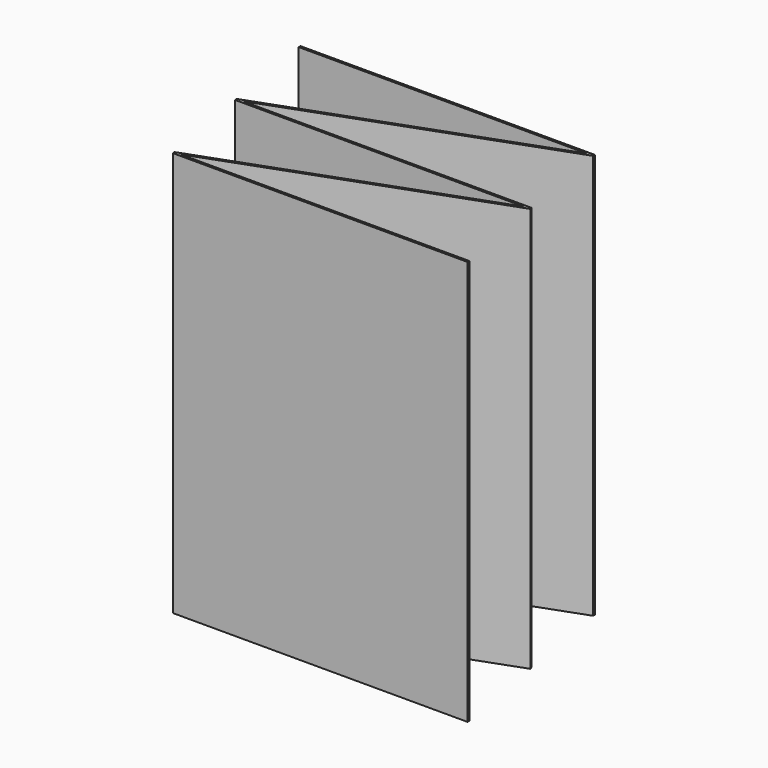
from build123d import *

# Parameters (mm, degrees)
F0_W     = 80
F0_H     = 110
F1_DEPTH = 0.6
F2_COUNT = 2
F2_ANGLE = 20
F3_COUNT = 2
F3_ANGLE = 20
F4_COUNT = 2
F4_ANGLE = 20
F5_COUNT = 2
F5_ANGLE = 20


with BuildPart() as f1:
    # F0 (on Front) → F1 (new body)
    with BuildSketch(Plane.XZ):
        Rectangle(F0_W, F0_H)
    extrude(amount=F1_DEPTH)


with BuildPart() as f2_1:
    # F2: instance of F1
    add(f1.part.rotate(Axis((-40, -0.6, 0), (0, 0, 1)), 1 * F2_ANGLE / (F2_COUNT - 1)))


with BuildPart() as f3_1:
    # F3: instance of F2_1
    add(f2_1.part.rotate(Axis((34.9701975769, 27.3254270385, 0), (0, 0, -1)), 1 * F3_ANGLE / (F3_COUNT - 1)))


with BuildPart() as f4_1:
    # F4: instance of F3_1
    add(f3_1.part.rotate(Axis((-45.0298024231, 27.3254270385, 0), (0, 0, 1)), 1 * F4_ANGLE / (F4_COUNT - 1)))


with BuildPart() as f5_1:
    # F5: instance of F4_1
    add(f4_1.part.rotate(Axis((30.3508193257, 54.1232229321, 0), (0, 0, -1)), 1 * F5_ANGLE / (F5_COUNT - 1)))


solid = Compound([f1.part, f2_1.part, f3_1.part, f4_1.part, f5_1.part])
